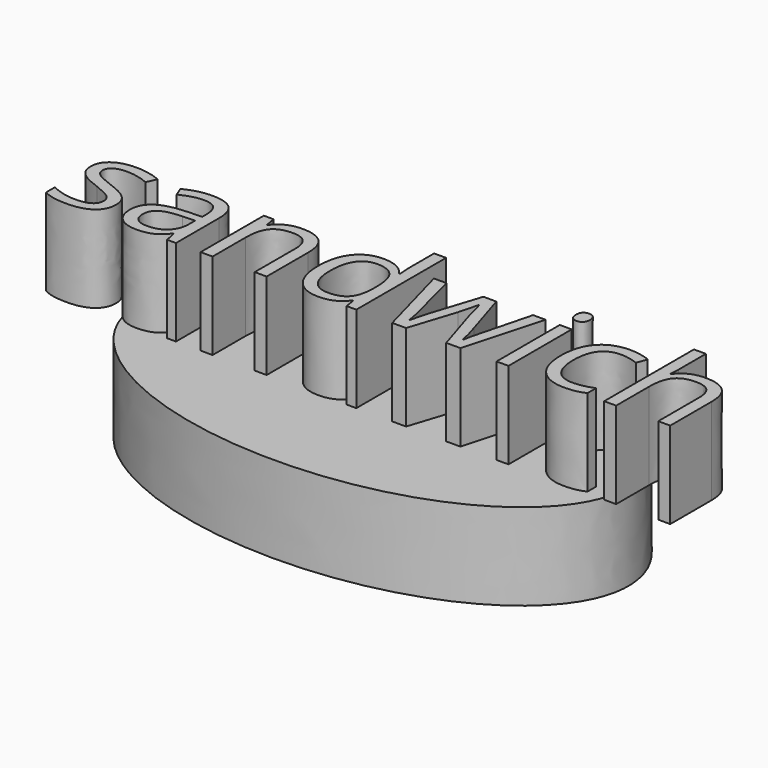
from build123d import *

# Parameters (mm, degrees)
F1_DEPTH     = 25.4
F2_TEXT_SIZE = 43.238090196
F3_DEPTH     = 25.4


# Not quite as in the source:
# - Text() gives the source's letters only with a copy of the font that has no kerning and outlines rounded to 1/6400 em; it was checked with that copy


with BuildPart() as f1:
    # F0 (on Top) → F1 (new body)
    with BuildSketch(Plane.XY):
        with BuildLine():
            add(Edge.make_bspline(
                [(-72.0287039876, 0), (-72.0287039876, -69.4017445183), (36.0143519938, -34.7008722591), (144.0574079752, 0), (36.0143519938, 34.7008722591), (-72.0287039876, 69.4017445183), (-72.0287039876, 0)],
                knots=[0, 0, 0, 2.0943951024, 2.0943951024, 4.1887902048, 4.1887902048, 6.2831853072, 6.2831853072, 6.2831853072], degree=2, weights=[1, 0.5, 1, 0.5, 1, 0.5, 1]))
        make_face()
    extrude(amount=F1_DEPTH)

    # F2 (on face) → F3 (join)
    with BuildSketch(Plane.XY.offset(25.4)):
        with Locations((-95.1132215559, -8.2259380724)):
            Text('sandwich', F2_TEXT_SIZE, font='Open Sans', text_align=(TextAlign.LEFT, TextAlign.BOTTOM))
    extrude(amount=F3_DEPTH)


solid = f1.part
